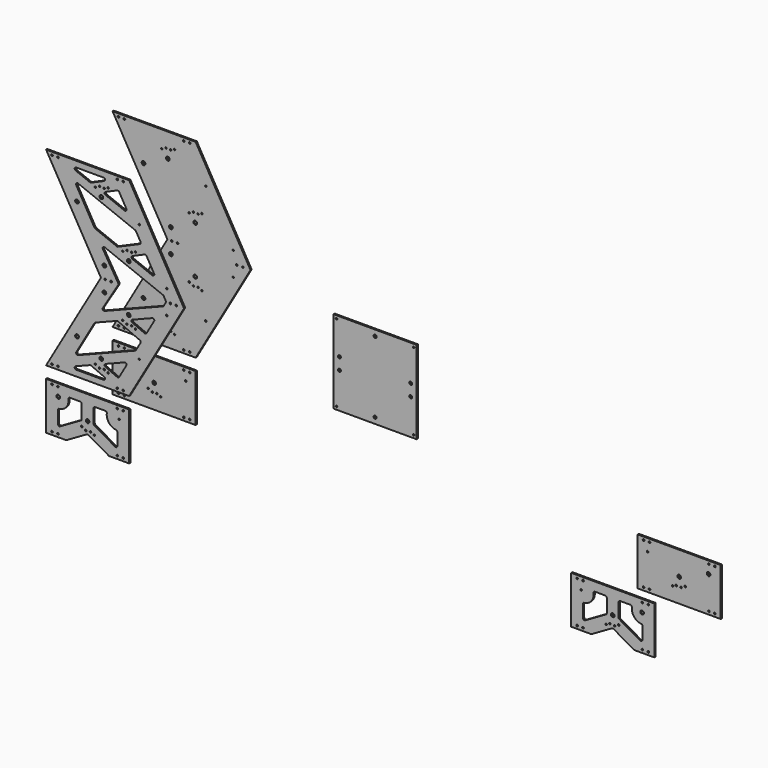
from build123d import *

# Parameters (mm, degrees)
F0_W      = 355.6
F0_H      = 355.6
F1_DEPTH  = 6.35
F2_D      = 6.7564
F2_DEPTH  = 26.0604
F2_TIP    = 2.0298273432
F3_R      = 6.35
F4_DEPTH  = 25.4
F6_DEPTH  = 6.35
F8_D      = 7.1374
F8_DEPTH  = 26.0604
F8_TIP    = 2.1442912911
F10_D     = 6.35
F10_DEPTH = 26.0604
F10_TIP   = 1.9077324654
F13_DEPTH = 25.4
F14_D     = 15.875
F14_DEPTH = 6.35
F14_TIP   = 4.7693311635
F16_D     = 15.875
F16_DEPTH = 6.35
F16_TIP   = 4.7693311635
F17_W     = 355.6
F17_H     = 203.2
F18_DEPTH = 6.35
F19_D     = 7.1374
F19_DEPTH = 26.0604
F19_TIP   = 2.1442912911
F21_D     = 6.7564
F21_DEPTH = 26.0604
F21_TIP   = 2.0298273432
F22_D     = 15.621
F25_DEPTH = 6.35


# Not quite as in the source:
# - a feature names something its author has since deleted; it is built from what else it names


with BuildPart() as f1:
    # F0 (on Front) → F1 (new body)
    with BuildSketch(Plane.XZ):
        with Locations((177.8, 177.8)):
            Rectangle(F0_W, F0_H)
    extrude(amount=F1_DEPTH)

    # F2
    with Locations(Plane(origin=(0, 0, 0), x_dir=(1, 0, 0), z_dir=(0, 1, 0))):
        with Locations((12.7, -342.9), (342.9, -342.9), (342.9, -12.7), (12.7, -12.7)):
            Hole(F2_D / 2, depth=F2_DEPTH)
            with Locations((0, 0, -(F2_DEPTH + F2_TIP / 2))):  # 118° drill point
                Cone(0, F2_D / 2, F2_TIP, mode=Mode.SUBTRACT)

    # F3 (on face) → F4 (cut)
    with BuildSketch(Plane.XZ.offset(6.35)):
        with Locations((25.4, 203.2)):
            Circle(F3_R)
        with Locations((177.8, 330.2)):
            Circle(F3_R)
        with Locations((330.2, 203.2)):
            Circle(F3_R)
        with Locations((25.4, 152.4)):
            Circle(F3_R)
        with Locations((330.2, 152.4)):
            Circle(F3_R)
        with Locations((177.8, 25.4)):
            Circle(F3_R)
    extrude(amount=-F4_DEPTH, mode=Mode.SUBTRACT)


with BuildPart() as f6:
    # F5 (on Front) → F6 (new body)
    with BuildSketch(Plane.XZ):
        Polygon((-945.8351493987, 0), (-590.2351493987, 0), (-355.6, 406.4), (-590.2351493987, 812.8), (-945.8351493987, 812.8), (-711.2, 406.4), align=None)
    extrude(amount=F6_DEPTH)

    # F8
    with Locations(Plane.XZ.offset(6.35)):
        with Locations((-895.0351493987, 800.1), (-641.0351493987, 800.1), (-667.7323484187, 406.4), (-413.7323484187, 406.4), (-641.0351493987, 12.7), (-895.0351493987, 12.7), (-920.4351493987, 12.7), (-615.6351493987, 12.7), (-615.6351493987, 800.1), (-920.4351493987, 800.1), (-693.1323484187, 406.4), (-388.3323484187, 406.4)):
            Hole(F8_D / 2, depth=F8_DEPTH)
            with Locations((0, 0, -(F8_DEPTH + F8_TIP / 2))):  # 118° drill point
                Cone(0, F8_D / 2, F8_TIP, mode=Mode.SUBTRACT)

    # F10
    with Locations(Plane.XZ.offset(6.35)):
        with Locations((-592.0587873497, 304.8), (-592.0587873497, 508), (-546.6969683742, 152.4), (-429.3793936748, 355.6), (-429.3793936748, 457.2), (-546.6969683742, 660.4), (-813.3969683742, 152.4), (-696.0793936748, 355.6), (-696.0793936748, 457.2), (-813.3969683742, 660.4), (-617.6111873497, 536.7274), (-599.7803873497, 545.6428), (-579.8921873497, 544.4998), (-563.1789873497, 551.6626), (-734.928762049, 739.9274), (-717.097962049, 748.8428), (-697.209762049, 747.6998), (-680.496562049, 754.8626), (-709.376362049, 711.2), (-617.6111873497, 276.0726), (-599.7803873497, 267.1572), (-579.8921873497, 268.3002), (-563.1789873497, 261.1374), (-709.376362049, 101.6), (-734.928762049, 72.8726), (-717.097962049, 63.9572), (-697.209762049, 65.1002), (-680.496562049, 57.9374)):
            Hole(F10_D / 2, depth=F10_DEPTH)
            with Locations((0, 0, -(F10_DEPTH + F10_TIP / 2))):  # 118° drill point
                Cone(0, F10_D / 2, F10_TIP, mode=Mode.SUBTRACT)


with BuildPart() as f11_1:
    # F11: copy of F6
    add(f6.part.moved(Location((0, -355.6, 0))))

    # F12 (on face) → F13 (cut)
    with BuildSketch(Plane.XZ.offset(361.95)):
        with BuildLine():
            Line((-602.2123596823, 701.5628652074), (-633.2825967243, 755.3780943674))
            ThreePointArc((-633.2825967243, 755.3780943674), (-636.7914340043, 758.2330787923), (-641.3103723061, 758.0279648036))
            Line((-641.3103723061, 758.0279648036), (-691.4544199928, 736.2609673383))
            ThreePointArc((-691.4544199928, 736.2609673383), (-695.2750048193, 730.3291357341), (-691.2567815249, 724.5293619322))
            Line((-691.2567815249, 724.5293619322), (-610.0424967962, 692.4811302374))
            ThreePointArc((-610.0424967962, 692.4811302374), (-602.902344106, 694.2413780445), (-602.2123596823, 701.5628652074))
        make_face()
        with BuildLine():
            ThreePointArc((-817.1879570156, 787.4), (-823.426156558, 782.2363247744), (-819.5188328155, 775.14326503))
            Line((-819.5188328155, 775.14326503), (-758.083859156, 750.9002112793))
            ThreePointArc((-758.083859156, 750.9002112793), (-755.6460221881, 750.457847155), (-753.2244690884, 750.9820758131))
            Line((-753.2244690884, 750.9820758131), (-697.3763970109, 775.2251295639))
            ThreePointArc((-697.3763970109, 775.2251295639), (-693.6875795652, 782.3412344347), (-699.9049112787, 787.4))
            Line((-699.9049112787, 787.4), (-817.1879570156, 787.4))
        make_face()
        with BuildLine():
            Line((-564.547261489, 633.5689317461), (-808.7102273018, 729.9188697626))
            ThreePointArc((-808.7102273018, 729.9188697626), (-815.850379992, 728.1586219555), (-816.5403644157, 720.8371347926))
            Line((-816.5403644157, 720.8371347926), (-738.7605543181, 586.1185519004))
            ThreePointArc((-738.7605543181, 586.1185519004), (-737.407780167, 584.4842750101), (-735.5921688039, 583.3868169305))
            Line((-735.5921688039, 583.3868169305), (-642.8574368523, 546.7924642785))
            ThreePointArc((-642.8574368523, 546.7924642785), (-640.4195998844, 546.3501001542), (-637.9980467847, 546.8743288123))
            Line((-637.9980467847, 546.8743288123), (-544.501876681, 587.4600212632))
            ThreePointArc((-544.5018766811, 587.4600212632), (-541.0004065239, 591.2944676653), (-541.5311296348, 596.4598916994))
            Line((-541.5311296348, 596.4598916994), (-561.3788759749, 630.8371967761))
            ThreePointArc((-561.3788759749, 630.8371967761), (-562.731650126, 632.4714736665), (-564.547261489, 633.5689317461))
        make_face()
        with BuildLine():
            Line((-445.933967684, 428.1246804227), (-695.0623699191, 526.4340453733))
            ThreePointArc((-695.0623699191, 526.4340453733), (-702.2550917448, 524.6120323303), (-702.8096133142, 517.2128780125))
            Line((-702.8096133142, 517.2128780125), (-637.028197289, 409.7144323908))
            ThreePointArc((-637.028197289, 409.7144323908), (-636.0945648843, 406.4), (-637.028197289, 403.0855676092))
            Line((-637.028197289, 403.0855676092), (-702.8096133142, 295.5871219875))
            ThreePointArc((-702.8096133142, 295.5871219875), (-702.2550917448, 288.1879676697), (-695.0623699191, 286.3659546267))
            Line((-695.0623699191, 286.3659546267), (-445.933967684, 384.6753195773))
            ThreePointArc((-445.933967684, 384.6753195773), (-444.118356321, 385.772777657), (-442.7655821698, 387.4070545473))
            Line((-442.7655821698, 387.4070545473), (-433.6330871047, 403.225))
            ThreePointArc((-433.6330871047, 403.225), (-432.7823484187, 406.4), (-433.6330871047, 409.575))
            Line((-433.6330871047, 409.575), (-442.7655821698, 425.3929454527))
            ThreePointArc((-442.7655821698, 425.3929454527), (-444.118356321, 427.0272223431), (-445.933967684, 428.1246804227))
        make_face()
        with BuildLine():
            Line((-642.8574368523, 266.0075357215), (-735.5921688039, 229.4131830695))
            ThreePointArc((-735.5921688039, 229.4131830695), (-737.407780167, 228.3157249899), (-738.7605543181, 226.6814480996))
            Line((-738.7605543181, 226.6814480996), (-816.5403644157, 91.9628652074))
            ThreePointArc((-816.5403644157, 91.9628652074), (-815.850379992, 84.6413780445), (-808.7102273018, 82.8811302374))
            Line((-808.7102273018, 82.8811302374), (-564.547261489, 179.2310682539))
            ThreePointArc((-564.547261489, 179.2310682539), (-562.731650126, 180.3285263335), (-561.3788759749, 181.9628032239))
            Line((-561.3788759749, 181.9628032239), (-541.5311296348, 216.3401083006))
            ThreePointArc((-541.5311296348, 216.3401083006), (-541.0004065239, 221.5055323347), (-544.5018766811, 225.3399787368))
            Line((-544.5018766811, 225.3399787368), (-637.9980467847, 265.9256711877))
            ThreePointArc((-637.9980467847, 265.9256711877), (-640.4195998844, 266.4498998458), (-642.8574368523, 266.0075357215))
        make_face()
        with BuildLine():
            Line((-758.083859156, 61.8997887207), (-819.5188328155, 37.65673497))
            ThreePointArc((-819.5188328155, 37.65673497), (-823.426156558, 30.5636752256), (-817.1879570156, 25.4))
            Line((-817.1879570156, 25.4), (-699.9049112787, 25.4))
            ThreePointArc((-699.9049112787, 25.4), (-693.6875795652, 30.4587655653), (-697.3763970109, 37.5748704361))
            Line((-697.3763970109, 37.5748704361), (-753.2244690884, 61.8179241869))
            ThreePointArc((-753.2244690884, 61.8179241869), (-755.6460221881, 62.342152845), (-758.083859156, 61.8997887207))
        make_face()
        with BuildLine():
            Line((-576.0303592212, 520.4216149314), (-491.4292029911, 487.036878914))
            ThreePointArc((-491.4292029911, 487.036878914), (-484.2890503009, 488.797126721), (-483.5990658772, 496.1186138839))
            Line((-483.5990658772, 496.1186138839), (-515.965022025, 552.1780943674))
            ThreePointArc((-515.965022025, 552.1780943674), (-519.473859305, 555.0330787923), (-523.9927976068, 554.8279648036))
            Line((-523.9927976068, 554.8279648036), (-576.2279976891, 532.1532203375))
            ThreePointArc((-576.2279976891, 532.1532203375), (-580.0485825156, 526.2213887333), (-576.0303592212, 520.4216149314))
        make_face()
        with BuildLine():
            Line((-515.965022025, 260.6219056326), (-483.5990658772, 316.6813861161))
            ThreePointArc((-483.5990658772, 316.6813861161), (-484.2890503009, 324.002873279), (-491.4292029911, 325.763121086))
            Line((-491.4292029911, 325.763121086), (-576.0303592212, 292.3783850686))
            ThreePointArc((-576.0303592212, 292.3783850686), (-580.0485825156, 286.5786112667), (-576.2279976891, 280.6467796625))
            Line((-576.2279976891, 280.6467796625), (-523.9927976068, 257.9720351964))
            ThreePointArc((-523.9927976068, 257.9720351964), (-519.473859305, 257.7669212077), (-515.965022025, 260.6219056326))
        make_face()
        with BuildLine():
            ThreePointArc((-691.2567815249, 88.2706380678), (-695.2750048193, 82.4708642659), (-691.4544199928, 76.5390326617))
            Line((-691.4544199928, 76.5390326617), (-641.3103723061, 54.7720351964))
            ThreePointArc((-641.3103723061, 54.7720351964), (-636.7914340043, 54.5669212077), (-633.2825967243, 57.4219056326))
            Line((-633.2825967243, 57.4219056326), (-602.2123596823, 111.2371347926))
            ThreePointArc((-602.2123596823, 111.2371347926), (-602.902344106, 118.5586219555), (-610.0424967962, 120.3188697626))
            Line((-610.0424967962, 120.3188697626), (-691.2567815249, 88.2706380678))
        make_face()
    extrude(amount=-F13_DEPTH, mode=Mode.SUBTRACT)

    # F16
    with Locations(Plane.XZ.offset(361.95)):
        with Locations((-813.3969683742, 660.4), (-709.376362049, 711.2), (-592.0587873497, 508), (-696.0793936748, 457.2), (-696.0793936748, 355.6), (-592.0587873497, 304.8), (-813.3969683742, 152.4), (-709.376362049, 101.6)):
            Hole(F16_D / 2, depth=F16_DEPTH)
            with Locations((0, 0, -(F16_DEPTH + F16_TIP / 2))):  # 118° drill point
                Cone(0, F16_D / 2, F16_TIP, mode=Mode.SUBTRACT)


with BuildPart() as f6_1:
    add(f6.part)

    # F14
    with Locations(Plane.XZ.offset(6.35)):
        with Locations((-709.376362049, 101.6), (-592.0587873497, 304.8), (-592.0587873497, 508), (-709.376362049, 711.2), (-813.3969683742, 152.4), (-696.0793936748, 355.6), (-696.0793936748, 457.2), (-813.3969683742, 660.4)):
            Hole(F14_D / 2, depth=F14_DEPTH)
            with Locations((0, 0, -(F14_DEPTH + F14_TIP / 2))):  # 118° drill point
                Cone(0, F14_D / 2, F14_TIP, mode=Mode.SUBTRACT)


with BuildPart() as f18:
    # F17 (on Front) → F18 (new body)
    with BuildSketch(Plane.XZ):
        with Locations((-768.0351493987, -152.4)):
            Rectangle(F17_W, F17_H)
    extrude(amount=F18_DEPTH)

    # F19
    with Locations(Plane(origin=(0, 0, 0), x_dir=(1, 0, 0), z_dir=(0, 1, 0))):
        with Locations((-920.4351493987, 63.5), (-895.0351493987, 63.5), (-641.0351493987, 63.5), (-615.6351493987, 63.5), (-615.6351493987, 241.3), (-641.0351493987, 241.3), (-920.4351493987, 241.3), (-895.0351493987, 241.3)):
            Hole(F19_D / 2, depth=F19_DEPTH)
            with Locations((0, 0, -(F19_DEPTH + F19_TIP / 2))):  # 118° drill point
                Cone(0, F19_D / 2, F19_TIP, mode=Mode.SUBTRACT)

    # F21
    with Locations(Plane.XZ.offset(6.35)):
        with Locations((-793.5875493987, -181.1274), (-775.7567493987, -190.0428), (-755.8685493987, -189.1284), (-739.6633493987, -196.1134), (-632.6531493987, -101.6)):
            Hole(F21_D / 2, depth=F21_DEPTH)
            with Locations((0, 0, -(F21_DEPTH + F21_TIP / 2))):  # 118° drill point
                Cone(0, F21_D / 2, F21_TIP, mode=Mode.SUBTRACT)

    # F22 (through all)
    with Locations(Plane.XZ.offset(6.35)):
        with Locations((-768.0351493987, -152.4), (-893.8921493987, -101.6)):
            Hole(F22_D / 2)


with BuildPart() as f23_1:
    # F23: copy of F18
    add(f18.part.moved(Location((0, -355.6, 0))))

    # F24 (on face) → F25 (cut)
    with BuildSketch(Plane.XZ.offset(361.95)):
        with BuildLine():
            ThreePointArc((-650.5601493987, -210.400738686), (-644.2101493987, -210.400738686), (-641.0351493987, -204.9014773719))
            Line((-641.0351493987, -204.9014773719), (-641.0351493987, -151.224961559))
            ThreePointArc((-641.0351493987, -151.224961559), (-641.8858880846, -148.049961559), (-644.2101493987, -145.725700245))
            ThreePointArc((-644.2101493987, -145.725700245), (-675.9807685513, -130.0357061549), (-686.0003237784, -96.048110345))
            ThreePointArc((-686.0003237784, -96.048110345), (-687.5360149765, -91.0515181726), (-692.2999682031, -88.9))
            Line((-692.2999682031, -88.9), (-736.2851493987, -88.9))
            ThreePointArc((-736.2851493987, -88.9), (-740.7752774592, -90.7598719395), (-742.6351493987, -95.25))
            Line((-742.6351493987, -95.25), (-742.6351493987, -153.575038441))
            ThreePointArc((-742.6351493987, -153.575038441), (-741.7844107127, -156.750038441), (-739.4601493987, -159.074299755))
            Line((-739.4601493987, -159.074299755), (-650.5601493987, -210.400738686))
        make_face()
        with BuildLine():
            Line((-793.4351493987, -153.575038441), (-793.4351493987, -95.25))
            ThreePointArc((-793.4351493987, -95.25), (-795.2950213381, -90.7598719395), (-799.7851493987, -88.9))
            Line((-799.7851493987, -88.9), (-843.7703305942, -88.9))
            ThreePointArc((-843.7703305942, -88.9), (-848.5342838209, -91.0515181726), (-850.0699750189, -96.048110345))
            ThreePointArc((-850.0699750189, -96.048110345), (-860.089530246, -130.0357061549), (-891.8601493987, -145.725700245))
            ThreePointArc((-891.8601493987, -145.725700245), (-894.1844107127, -148.049961559), (-895.0351493987, -151.224961559))
            Line((-895.0351493987, -151.224961559), (-895.0351493987, -204.9014773719))
            ThreePointArc((-895.0351493987, -204.9014773719), (-891.8601493987, -210.400738686), (-885.5101493987, -210.400738686))
            Line((-885.5101493987, -210.400738686), (-796.6101493987, -159.074299755))
            ThreePointArc((-796.6101493987, -159.074299755), (-794.2858880846, -156.750038441), (-793.4351493987, -153.575038441))
        make_face()
        with BuildLine():
            Line((-771.2101493987, -203.0683902673), (-857.952762539, -253.149261314))
            ThreePointArc((-857.952762539, -253.149261314), (-859.4842616026, -253.7836289969), (-861.127762539, -254))
            Line((-861.127762539, -254), (-674.9425362584, -254))
            ThreePointArc((-674.9425362584, -254), (-676.5860371948, -253.7836289969), (-678.1175362584, -253.149261314))
            Line((-678.1175362584, -253.149261314), (-764.8601493987, -203.0683902673))
            ThreePointArc((-764.8601493987, -203.0683902673), (-768.0351493987, -202.2176515813), (-771.2101493987, -203.0683902673))
        make_face()
    extrude(amount=-F25_DEPTH, mode=Mode.SUBTRACT)


with BuildPart() as f26_1:
    # F26: instance of F18
    add(f18.part.mirror(Plane(origin=(355.6, -3.175, 177.8), x_dir=(0, 1, 0), z_dir=(1, 0, 0))))


with BuildPart() as f27_1:
    # F27: instance of F23_1
    add(f23_1.part.mirror(Plane(origin=(355.6, -3.175, 177.8), x_dir=(0, 1, 0), z_dir=(1, 0, 0))))


solid = Compound([f1.part, f11_1.part, f6_1.part, f18.part, f23_1.part, f26_1.part, f27_1.part])
